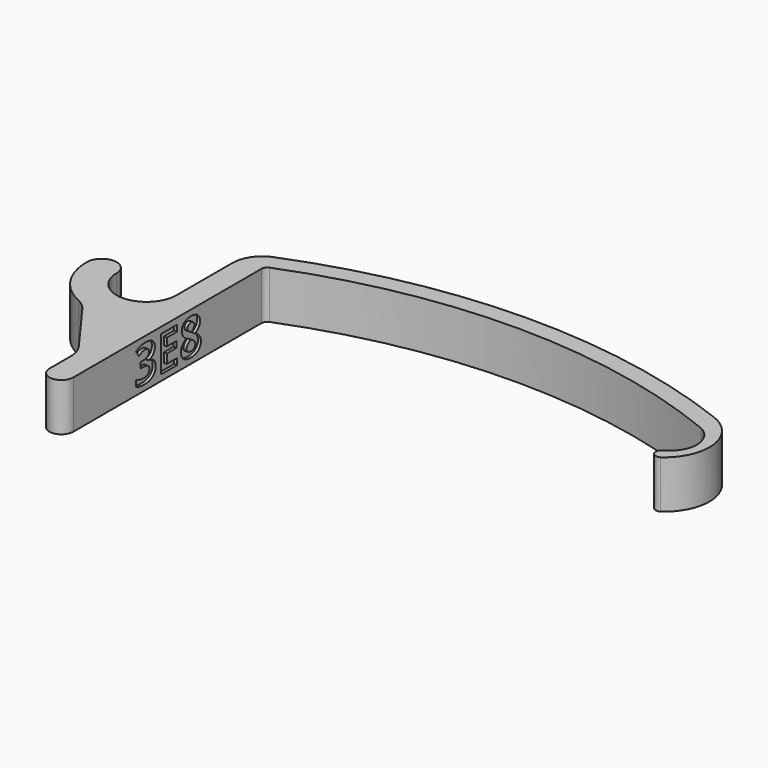
from build123d import *

# Parameters (mm, degrees)
F1_DEPTH     = 8
F2_TEXT_SIZE = 8.3333333333
F3_DEPTH     = 0.5
F4_T1_DEPTH  = 8
F5_R         = 5
F6_R         = 1


# Not quite as in the source:
# - a fillet or chamfer that OpenCascade refuses, or shapes differently, is made with other operations: its cross-section is extruded or revolved along the edge and cut away or added
# - Text() gives the source's letters only with a copy of the font that has no kerning and outlines rounded to 1/6400 em; it was checked with that copy


with BuildPart() as f1:
    # F0 (on Top) → F1 (new body)
    with BuildSketch(Plane.XY):
        with BuildLine():
            ThreePointArc((-36.5, 40), (0, 47.129259489), (36.5, 40))
            ThreePointArc((36.5, 40), (38.972135955, 36), (36.5, 32))
            ThreePointArc((36.5, 32), (36.1339745962, 30.6339745962), (37.5, 30.2679491924))
            ThreePointArc((37.5, 30.2679491924), (40.6592248075, 37.3527125473), (35.8867527428, 43.468109801))
            ThreePointArc((35.8867527428, 43.468109801), (-2.4959663869, 50.0981053951), (-40.5, 41.5609279633))
            Line((-40.5, 41.5609279633), (-40.5, 26.5609279633))
            ThreePointArc((-40.5, 26.5609279633), (-45.5, 21.5609279633), (-50.5, 26.5609279633))
            ThreePointArc((-50.5, 26.5609279633), (-53, 29.0609279633), (-55.5, 26.5609279633))
            ThreePointArc((-55.5, 26.5609279633), (-50.5, 17.9006739255), (-40.5, 17.9006739255))
            Line((-40.5, 17.9006739255), (-40.5, 0))
            ThreePointArc((-40.5, 0), (-38.5, -2), (-36.5, 0))
            Line((-36.5, 0), (-36.5, 40))
        make_face()
    extrude(amount=F1_DEPTH)

    # F2 (on face) → F3 (cut)
    with BuildSketch(Plane.YZ.offset(-36.5)):
        with Locations((12.7845052083, 1)):
            Text('3E8', F2_TEXT_SIZE, font='Open Sans', font_style=FontStyle.BOLD, text_align=(TextAlign.LEFT, TextAlign.BOTTOM))
    extrude(amount=-F3_DEPTH, mode=Mode.SUBTRACT)

    # F4: chamfer of 20 on 1 edges, made by hand

    # F4_s2 → F4_t1 (join)
    with BuildSketch(Plane.XY):
        with BuildLine():
            Line((-49.0104596448, 17.6796557771), (-40.0280161282, 5.3867164622))
            Line((-40.0280161282, 5.3867164622), (-39.6280161282, 5.3867164622))
            ThreePointArc((-39.6280161282, 5.3867164622), (-40.1, 11.6436951938), (-40.1, 17.9006739255))
            Line((-40.1, 17.9006739255), (-40.7, 18.247084087))
            ThreePointArc((-40.7, 18.247084087), (-44.6877382701, 16.9953526601), (-48.8889206138, 18.0607440398))
            Line((-48.8889206138, 18.0607440398), (-49.0104596448, 17.6796557771))
        make_face()
    extrude(amount=F4_T1_DEPTH)

    # F5
    f5_edges = [f1.edges().sort_by_distance(p)[0] for p in [
        (-40.5, 41.560928, 4),
        (-48.538476, 17.033721, 4),
        (-40.5, 6.032651, 4),
    ]]
    fillet(f5_edges, radius=F5_R)

    # F6
    f6_edges = [f1.edges().sort_by_distance(p)[0] for p in [
        (-36.5, 40, 4),
    ]]
    fillet(f6_edges, radius=F6_R)


solid = f1.part
